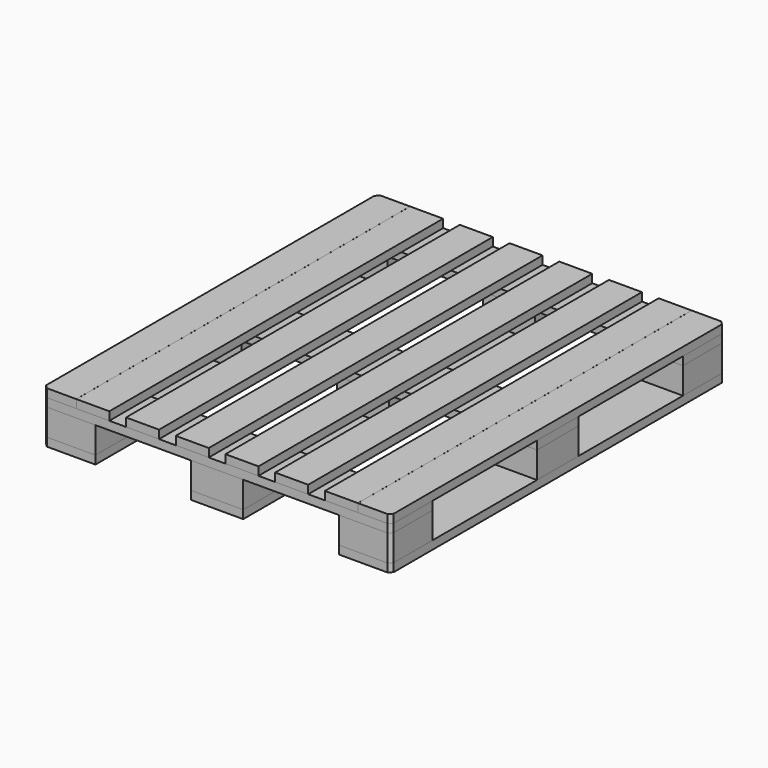
from build123d import *

# Parameters (mm, degrees)
F0_W        = 95
F0_H        = 800
F0_H_2      = 400
F1_DEPTH    = 24
F0_W_2      = 94.9
F2_W        = 1000
F2_H        = 150
F3_DEPTH    = 24
F5_W        = 150
F5_H        = 150
F6_DEPTH    = 76
F8_W        = 150
F8_H        = 1200
F9_DEPTH    = 24
F10_SIZE    = 10
F10_2_SIZE  = 10
F10_3_SIZE  = 10
F10_4_SIZE  = 10
F10_5_SIZE  = 10
F10_6_SIZE  = 10
F10_7_SIZE  = 10
F10_8_SIZE  = 10
F10_9_SIZE  = 10
F10_10_SIZE = 10


# Not quite as in the source:
# - a feature names something its author has since deleted; it is built from what else it names


with BuildPart() as f1:
    # F0 (on Top) → F1 (new body)
    with BuildSketch(Plane.XY):
        with Locations((47.5, 400)):
            Rectangle(F0_W, F0_H)
        with Locations((47.5, 1000)):
            Rectangle(F0_W, F0_H_2)
    extrude(amount=F1_DEPTH)

    # F10#3
    f10_3_edges = [f1.edges().sort_by_distance(p)[0] for p in [
        (0, 0, 12),
        (0, 1200, 12),
    ]]
    chamfer(f10_3_edges, length=F10_3_SIZE)


with BuildPart() as f1b:
    # F0 (on Top) → F1, piece 2 (new body)
    with BuildSketch(Plane.XY):
        with Locations((952.5, 1000)):
            Rectangle(F0_W, F0_H_2)
        with Locations((952.5, 400)):
            Rectangle(F0_W, F0_H)
    extrude(amount=F1_DEPTH)

    # F10#7
    f10_7_edges = [f1b.edges().sort_by_distance(p)[0] for p in [
        (1000, 0, 12),
        (1000, 1200, 12),
    ]]
    chamfer(f10_7_edges, length=F10_7_SIZE)


with BuildPart() as f1c:
    # F0 (on Top) → F1, piece 3 (new body)
    with BuildSketch(Plane.XY):
        with Locations((857.45, 1000)):
            Rectangle(F0_W_2, F0_H_2)
        with Locations((857.45, 400)):
            Rectangle(F0_W_2, F0_H)
    extrude(amount=F1_DEPTH)


with BuildPart() as f1d:
    # F0 (on Top) → F1, piece 4 (new body)
    with BuildSketch(Plane.XY):
        with Locations((714.5, 1000)):
            Rectangle(F0_W, F0_H_2)
        with Locations((714.5, 400)):
            Rectangle(F0_W, F0_H)
    extrude(amount=F1_DEPTH)


with BuildPart() as f1e:
    # F0 (on Top) → F1, piece 5 (new body)
    with BuildSketch(Plane.XY):
        with Locations((571.5, 1000)):
            Rectangle(F0_W, F0_H_2)
        with Locations((571.5, 400)):
            Rectangle(F0_W, F0_H)
    extrude(amount=F1_DEPTH)


with BuildPart() as f1f:
    # F0 (on Top) → F1, piece 6 (new body)
    with BuildSketch(Plane.XY):
        with Locations((428.5, 1000)):
            Rectangle(F0_W, F0_H_2)
        with Locations((428.5, 400)):
            Rectangle(F0_W, F0_H)
    extrude(amount=F1_DEPTH)


with BuildPart() as f1g:
    # F0 (on Top) → F1, piece 7 (new body)
    with BuildSketch(Plane.XY):
        with Locations((285.5, 1000)):
            Rectangle(F0_W, F0_H_2)
        with Locations((285.5, 400)):
            Rectangle(F0_W, F0_H)
    extrude(amount=F1_DEPTH)


with BuildPart() as f1h:
    # F0 (on Top) → F1, piece 8 (new body)
    with BuildSketch(Plane.XY):
        with Locations((142.55, 1000)):
            Rectangle(F0_W_2, F0_H_2)
        with Locations((142.55, 400)):
            Rectangle(F0_W_2, F0_H)
    extrude(amount=F1_DEPTH)


with BuildPart() as f3:
    # F2 (on Top) → F3 (new body)
    with BuildSketch(Plane.XY):
        with Locations((500, 75)):
            Rectangle(F2_W, F2_H)
    extrude(amount=-F3_DEPTH)

    # F10#2
    f10_2_edges = [f3.edges().sort_by_distance(p)[0] for p in [
        (0, 0, -12),
        (1000, 0, -12),
    ]]
    chamfer(f10_2_edges, length=F10_2_SIZE)


with BuildPart() as f3b:
    # F2 (on Top) → F3, piece 2 (new body)
    with BuildSketch(Plane.XY):
        with Locations((500, 600)):
            Rectangle(F2_W, F2_H)
    extrude(amount=-F3_DEPTH)


with BuildPart() as f3c:
    # F2 (on Top) → F3, piece 3 (new body)
    with BuildSketch(Plane.XY):
        with Locations((500, 1125)):
            Rectangle(F2_W, F2_H)
    extrude(amount=-F3_DEPTH)

    # F10#8
    f10_8_edges = [f3c.edges().sort_by_distance(p)[0] for p in [
        (1000, 1200, -12),
        (0, 1200, -12),
    ]]
    chamfer(f10_8_edges, length=F10_8_SIZE)


with BuildPart() as f6:
    # F5 (on offset) → F6 (new body)
    with BuildSketch(Plane.XY.offset(-24)):
        with Locations((75, 75)):
            Rectangle(F5_W, F5_H)
    extrude(amount=-F6_DEPTH)

    # F10
    f10_edges = [f6.edges().sort_by_distance(p)[0] for p in [
        (0, 0, -62),
    ]]
    chamfer(f10_edges, length=F10_SIZE)


with BuildPart() as f6b:
    # F5 (on offset) → F6, piece 2 (new body)
    with BuildSketch(Plane.XY.offset(-24)):
        with Locations((75, 600)):
            Rectangle(F5_W, F5_H)
    extrude(amount=-F6_DEPTH)


with BuildPart() as f6c:
    # F5 (on offset) → F6, piece 3 (new body)
    with BuildSketch(Plane.XY.offset(-24)):
        with Locations((75, 1125)):
            Rectangle(F5_W, F5_H)
    extrude(amount=-F6_DEPTH)

    # F10#10
    f10_10_edges = [f6c.edges().sort_by_distance(p)[0] for p in [
        (0, 1200, -62),
    ]]
    chamfer(f10_10_edges, length=F10_10_SIZE)


with BuildPart() as f6d:
    # F5 (on offset) → F6, piece 4 (new body)
    with BuildSketch(Plane.XY.offset(-24)):
        with Locations((500, 75)):
            Rectangle(F5_W, F5_H)
    extrude(amount=-F6_DEPTH)


with BuildPart() as f6e:
    # F5 (on offset) → F6, piece 5 (new body)
    with BuildSketch(Plane.XY.offset(-24)):
        with Locations((500, 1125)):
            Rectangle(F5_W, F5_H)
    extrude(amount=-F6_DEPTH)


with BuildPart() as f6f:
    # F5 (on offset) → F6, piece 6 (new body)
    with BuildSketch(Plane.XY.offset(-24)):
        with Locations((925, 75)):
            Rectangle(F5_W, F5_H)
    extrude(amount=-F6_DEPTH)

    # F10#6
    f10_6_edges = [f6f.edges().sort_by_distance(p)[0] for p in [
        (1000, 0, -62),
    ]]
    chamfer(f10_6_edges, length=F10_6_SIZE)


with BuildPart() as f6g:
    # F5 (on offset) → F6, piece 7 (new body)
    with BuildSketch(Plane.XY.offset(-24)):
        with Locations((925, 1125)):
            Rectangle(F5_W, F5_H)
    extrude(amount=-F6_DEPTH)

    # F10#9
    f10_9_edges = [f6g.edges().sort_by_distance(p)[0] for p in [
        (1000, 1200, -62),
    ]]
    chamfer(f10_9_edges, length=F10_9_SIZE)


with BuildPart() as f6h:
    # F5 (on offset) → F6, piece 8 (new body)
    with BuildSketch(Plane.XY.offset(-24)):
        with Locations((925, 600)):
            Rectangle(F5_W, F5_H)
    extrude(amount=-F6_DEPTH)


with BuildPart() as f6i:
    # F5 (on offset) → F6, piece 9 (new body)
    with BuildSketch(Plane.XY.offset(-24)):
        with Locations((500, 600)):
            Rectangle(F5_W, F5_H)
    extrude(amount=-F6_DEPTH)


with BuildPart() as f9:
    # F8 (on offset) → F9 (new body)
    with BuildSketch(Plane.XY.offset(-100)):
        with Locations((75, 600)):
            Rectangle(F8_W, F8_H)
    extrude(amount=-F9_DEPTH)

    # F10#4
    f10_4_edges = [f9.edges().sort_by_distance(p)[0] for p in [
        (0, 0, -112),
        (0, 1200, -112),
    ]]
    chamfer(f10_4_edges, length=F10_4_SIZE)


with BuildPart() as f9b:
    # F8 (on offset) → F9, piece 2 (new body)
    with BuildSketch(Plane.XY.offset(-100)):
        with Locations((500, 600)):
            Rectangle(F8_W, F8_H)
    extrude(amount=-F9_DEPTH)


with BuildPart() as f9c:
    # F8 (on offset) → F9, piece 3 (new body)
    with BuildSketch(Plane.XY.offset(-100)):
        with Locations((925, 600)):
            Rectangle(F8_W, F8_H)
    extrude(amount=-F9_DEPTH)

    # F10#5
    f10_5_edges = [f9c.edges().sort_by_distance(p)[0] for p in [
        (1000, 0, -112),
        (1000, 1200, -112),
    ]]
    chamfer(f10_5_edges, length=F10_5_SIZE)


solid = Compound([f1.part, f1b.part, f1c.part, f1d.part, f1e.part, f1f.part, f1g.part, f1h.part, f3.part, f3b.part, f3c.part, f6.part, f6b.part, f6c.part, f6d.part, f6e.part, f6f.part, f6g.part, f6h.part, f6i.part, f9.part, f9b.part, f9c.part])
